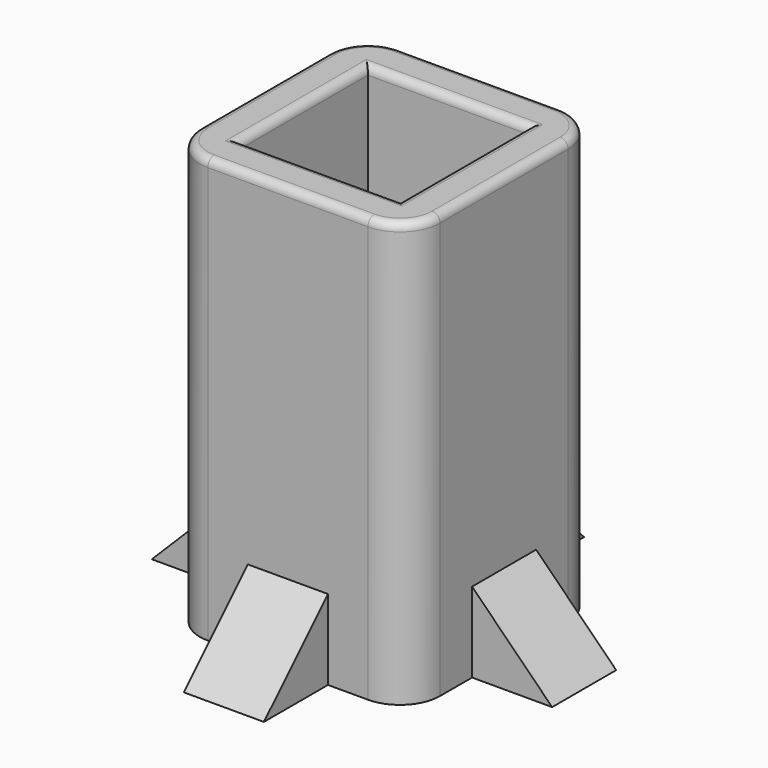
from build123d import *

# Parameters (mm, degrees)
F0_W            = 30
F0_H            = 30
F1_DEPTH        = 3
F2_W            = 30
F2_H            = 30
F2_W_2          = 20
F2_H_2          = 20
F3_DEPTH        = 50
F4_R            = 5
F5_R            = 1
F7_DEPTH        = 5
F7_DEPTH_BACK   = 5
F7_COPIES_COUNT = 4


# Not quite as in the source:
# - a pattern or mirror of a feature is missing from the dataset's text; its kind, count and spacing are read off the source's solid


with BuildPart() as f1:
    # F0 (on Top) → F1 (new body)
    with BuildSketch(Plane.XY):
        Rectangle(F0_W, F0_H)
    extrude(amount=F1_DEPTH)

    # F2 (on face) → F3 (join)
    with BuildSketch(Plane.XY.offset(3)):
        Rectangle(F2_W, F2_H)
        Rectangle(F2_W_2, F2_H_2, mode=Mode.SUBTRACT)
    extrude(amount=F3_DEPTH)

    # F4
    f4_edges = [f1.edges().sort_by_distance(p)[0] for p in [
        (-15, -15, 26.5),
        (-15, 15, 26.5),
        (15, 15, 26.5),
        (15, -15, 26.5),
    ]]
    fillet(f4_edges, radius=F4_R)

    # F5
    f5_edges = [f1.edges().sort_by_distance(p)[0] for p in [
        (15, 0, 53),
        (13.535534, -13.535534, 53),
        (13.535534, 13.535534, 53),
        (0, -15, 53),
        (0, 15, 53),
        (-13.535534, -13.535534, 53),
        (-13.535534, 13.535534, 53),
        (-15, 0, 53),
        (0, 10, 53),
        (10, 0, 53),
        (0, -10, 53),
        (-10, 0, 53),
    ]]
    fillet(f5_edges, radius=F5_R)

    # F6 (on Front) → F7 (join, two sides)
    with BuildSketch(Plane.XZ) as f7_sk:
        Polygon((15, 10), (15, 0), (25, 0), align=None)
    f7 = extrude(amount=F7_DEPTH) + extrude(f7_sk.sketch, amount=-F7_DEPTH_BACK)

    # F7_copies: F7 ×4 about axis
    f7_copies_axis = Axis((0, 0, 0), (0, 0, 1))
    for i in range(1, F7_COPIES_COUNT):
        add(f7.rotate(f7_copies_axis, i * 360 / F7_COPIES_COUNT))


solid = f1.part
